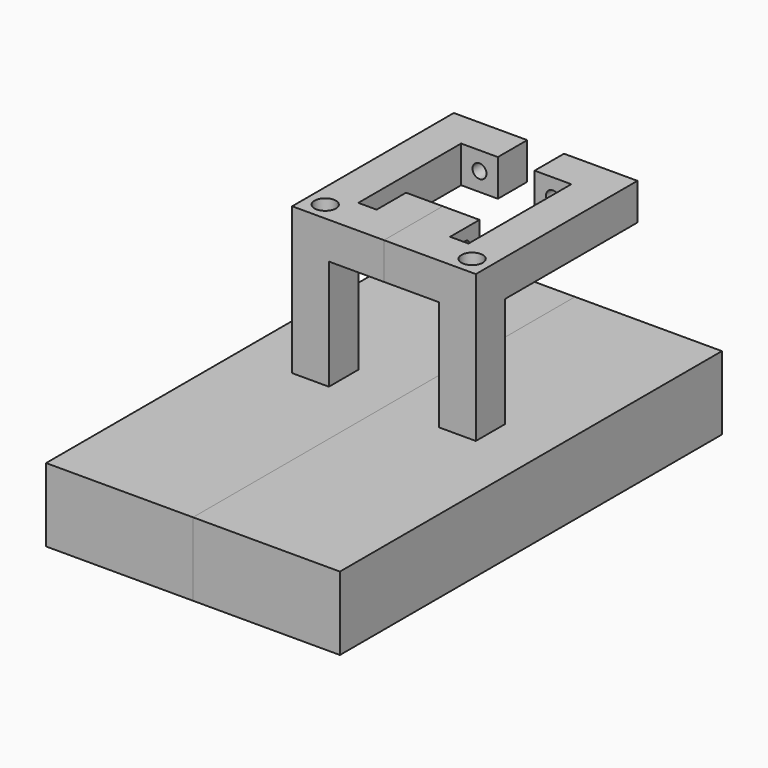
from build123d import *

# Parameters (mm, degrees)
F0_W      = 20
F0_H      = 65
F0_W_2    = 5
F0_H_2    = 5
F1_DEPTH  = 10
F2_DEPTH  = 30
F3_W      = 5
F3_H      = 5
F4_DEPTH  = 7.5
F5_W      = 5
F5_H      = 5
F6_DEPTH  = 22.5
F7_R      = 1.45
F8_DEPTH  = 2.5
F9_R      = 0.95
F10_DEPTH = 5
F11_R     = 0.95
F12_DEPTH = 5
F13_W     = 5
F13_H     = 5
F14_DEPTH = 5
F15_W     = 5
F15_H     = 5
F16_DEPTH = 5
F18_R     = 0.95
F19_DEPTH = 5
F20_R     = 0.95
F21_DEPTH = 5


with BuildPart() as f1:
    # F0 (on Top) → F1 (new body)
    with BuildSketch(Plane.XY):
        with Locations((-0.8371751755, 12.2564576566)):
            Rectangle(F0_W, F0_H)
        with Locations((-0.8371751755, 14.7564576566)):
            Rectangle(F0_W_2, F0_H_2, mode=Mode.SUBTRACT)
    extrude(amount=F1_DEPTH)

    # F0 (on Top) → F2 (join)
    with BuildSketch(Plane.XY):
        with Locations((-0.8371751755, 14.7564576566)):
            Rectangle(F0_W_2, F0_H_2)
    extrude(amount=F2_DEPTH)

    # F3 (on face) → F4 (join)
    with BuildSketch(Plane.YZ.offset(1.6628248245)):
        with Locations((14.7564576566, 27.5)):
            Rectangle(F3_W, F3_H)
    extrude(amount=F4_DEPTH)

    # F5 (on face) → F6 (join)
    with BuildSketch(Plane(origin=(0, 17.2564576566, 0), x_dir=(-1, 0, 0), z_dir=(0, 1, 0))):
        with Locations((0.8371751755, 27.5)):
            Rectangle(F5_W, F5_H)
    extrude(amount=F6_DEPTH)

    # F7 (on face) → F8 (cut)
    with BuildSketch(Plane.XY.offset(30)):
        with Locations((-0.8371751755, 14.7564576566)):
            Circle(F7_R)
    extrude(amount=-F8_DEPTH, mode=Mode.SUBTRACT)

    # F9 (on face) → F10 (cut)
    with BuildSketch(Plane(origin=(0, 39.7564576566, 0), x_dir=(-1, 0, 0), z_dir=(0, 1, 0))):
        with Locations((0.8371751755, 27.5)):
            Circle(F9_R)
    extrude(amount=-F10_DEPTH, mode=Mode.SUBTRACT)

    # F11 (on face) → F12 (cut)
    with BuildSketch(Plane.YZ.offset(9.1628248245)):
        with Locations((14.7564576566, 27.5)):
            Circle(F11_R)
    extrude(amount=-F12_DEPTH, mode=Mode.SUBTRACT)

    # F13 (on face) → F14 (join)
    with BuildSketch(Plane(origin=(0, 17.2564576566, 0), x_dir=(-1, 0, 0), z_dir=(0, 1, 0))):
        with Locations((-6.6628248245, 27.5)):
            Rectangle(F13_W, F13_H)
    extrude(amount=F14_DEPTH)

    # F15 (on face) → F16 (join)
    with BuildSketch(Plane.YZ.offset(1.6628248245)):
        with Locations((37.2564576566, 27.5)):
            Rectangle(F15_W, F15_H)
    extrude(amount=F16_DEPTH)

    # F17: union 

    # F18 (on face) → F19 (cut)
    with BuildSketch(Plane(origin=(0, 39.7564576566, 0), x_dir=(-1, 0, 0), z_dir=(0, 1, 0))):
        with Locations((-4.1628248245, 27.5)):
            Circle(F18_R)
    extrude(amount=-F19_DEPTH, mode=Mode.SUBTRACT)

    # F20 (on face) → F21 (cut)
    with BuildSketch(Plane.YZ.offset(9.1628248245)):
        with Locations((19.7564576566, 27.5)):
            Circle(F20_R)
    extrude(amount=-F21_DEPTH, mode=Mode.SUBTRACT)


with BuildPart() as f22_1:
    # F22: instance of F1
    add(f1.part.mirror(Plane(origin=(9.1628248245, 12.2564576566, 5), x_dir=(0, 1, 0), z_dir=(1, 0, 0))))


solid = Compound([f1.part, f22_1.part])
